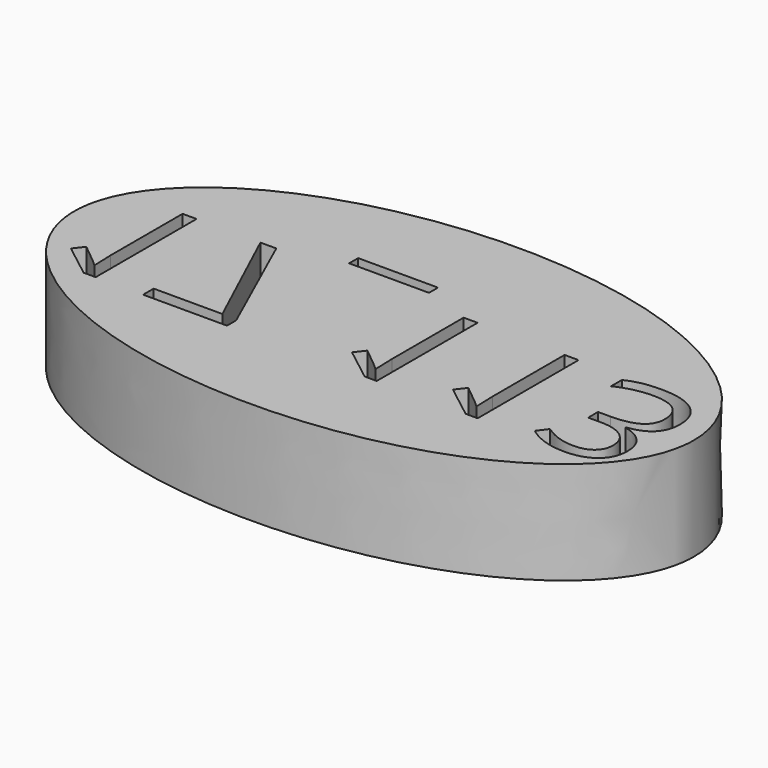
from build123d import *

# Parameters (mm, degrees)
F1_DEPTH     = 25.4
F2_TEXT_SIZE = 43.7397794384
F3_DEPTH     = 25.4


# Not quite as in the source:
# - Text() gives the source's letters only with a copy of the font that has no kerning and outlines rounded to 1/6400 em; it was checked with that copy


with BuildPart() as f1:
    # F0 (on Top) → F1 (new body)
    with BuildSketch(Plane.XY):
        with BuildLine():
            add(Edge.make_bspline(
                [(76.7747461796, 0), (76.7747461796, 72.2729841788), (-38.3873730898, 36.1364920894), (-153.5494923592, 0), (-38.3873730898, -36.1364920894), (76.7747461796, -72.2729841788), (76.7747461796, 0)],
                knots=[0, 0, 0, 2.0943951024, 2.0943951024, 4.1887902048, 4.1887902048, 6.2831853072, 6.2831853072, 6.2831853072], degree=2, weights=[1, 0.5, 1, 0.5, 1, 0.5, 1]))
        make_face()
    extrude(amount=F1_DEPTH)

    # F2 (on face) → F3 (cut)
    with BuildSketch(Plane(origin=(0, 0, 0), x_dir=(1, 0, 0), z_dir=(0, 0, -1))):
        with Locations((-71.5360300931, -12.2719124845)):
            Text('17_113', F2_TEXT_SIZE, font='Open Sans', text_align=(TextAlign.LEFT, TextAlign.BOTTOM))
    extrude(amount=-F3_DEPTH, mode=Mode.SUBTRACT)


solid = f1.part
